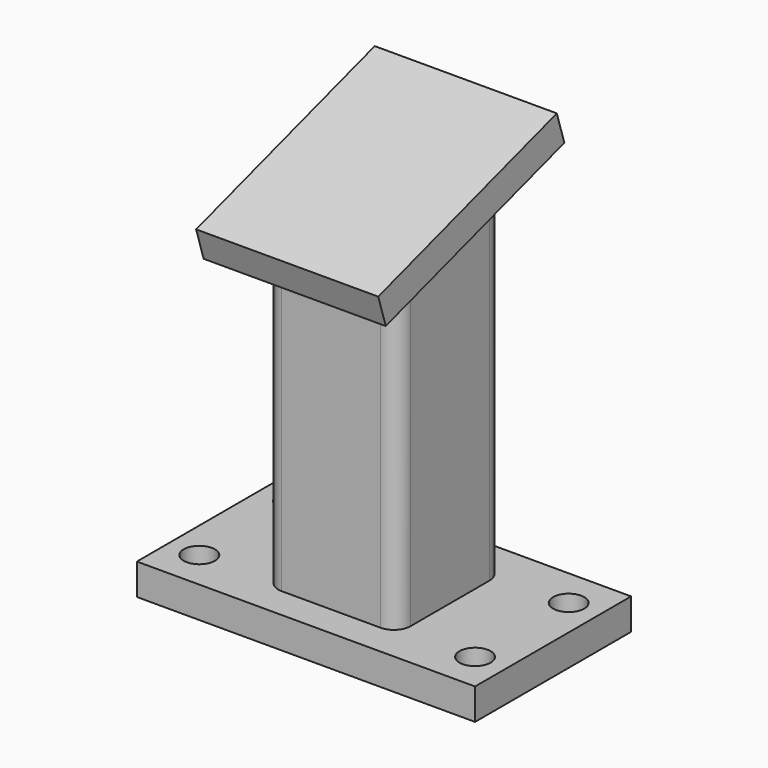
from build123d import *

# Parameters (mm, degrees)
F0_W     = 130
F0_H     = 75
F1_DEPTH = 12
F3_DEPTH = 136
F5_D     = 12
F7_DEPTH = 50.8
F8_W     = 70
F8_H     = 90
F9_DEPTH = 12


with BuildPart() as f1:
    # F0 (on Top) → F1 (new body)
    with BuildSketch(Plane.XY):
        Rectangle(F0_W, F0_H)
    extrude(amount=-F1_DEPTH)

    # F2 (on face) → F3 (join)
    with BuildSketch(Plane.XY):
        with BuildLine():
            Line((-19.05, -25.4), (19.05, -25.4))
            ThreePointArc((19.05, -25.4), (23.5401280605, -23.5401280605), (25.4, -19.05))
            Line((25.4, -19.05), (25.4, 19.05))
            ThreePointArc((25.4, 19.05), (23.5401280605, 23.5401280605), (19.05, 25.4))
            Line((19.05, 25.4), (-19.05, 25.4))
            ThreePointArc((-19.05, 25.4), (-23.5401280605, 23.5401280605), (-25.4, 19.05))
            Line((-25.4, 19.05), (-25.4, -19.05))
            ThreePointArc((-25.4, -19.05), (-23.5401280605, -23.5401280605), (-19.05, -25.4))
        make_face()
        with BuildLine():
            Line((-12.7, 19.05), (12.7, 19.05))
            ThreePointArc((12.7, 19.05), (17.1901280605, 17.1901280605), (19.05, 12.7))
            Line((19.05, 12.7), (19.05, -12.7))
            ThreePointArc((19.05, -12.7), (17.1901280605, -17.1901280605), (12.7, -19.05))
            Line((12.7, -19.05), (-12.7, -19.05))
            ThreePointArc((-12.7, -19.05), (-17.1901280605, -17.1901280605), (-19.05, -12.7))
            Line((-19.05, -12.7), (-19.05, 12.7))
            ThreePointArc((-19.05, 12.7), (-17.1901280605, 17.1901280605), (-12.7, 19.05))
        make_face(mode=Mode.SUBTRACT)
    extrude(amount=F3_DEPTH)

    # F5 (through all)
    with Locations(Plane.XY):
        with Locations((-53, 22.5), (53, 22.5), (53, -22.5), (-53, -22.5)):
            Hole(F5_D / 2)

    # F6 (on face) → F7 (cut)
    with BuildSketch(Plane.YZ.offset(25.4)):
        Polygon((-19.05, 136), (-25.4, 136), (-25.4, 119.9340696072), (-19.05, 121.9423109063), align=None)
        Polygon((19.05, 136), (-19.05, 136), (-19.05, 121.9423109063), (19.05, 133.9917587009), align=None)
        Polygon((25.4, 136), (19.05, 136), (19.05, 133.9917587009), align=None)
    extrude(amount=-F7_DEPTH, mode=Mode.SUBTRACT)

    # F8 (on face) → F9 (join)
    with BuildSketch(Plane(origin=(0, -36.7908585502, 116.331614084), x_dir=(1, 0, 0), z_dir=(0, -0.3015379599, 0.9534541723))):
        with Locations((0, 38.5869186148)):
            Rectangle(F8_W, F8_H)
        with BuildLine():
            Line((25.4, 58.5669035507), (25.4, 18.6069336789))
            add(Edge.make_bspline(
                [(25.4, 18.6069336789), (25.4, 11.9469387003), (19.05, 11.9469387003)],
                knots=[4.7123889804, 4.7123889804, 4.7123889804, 6.2831853072, 6.2831853072, 6.2831853072], degree=2, weights=[1, 0.7071067812, 1]))
            Line((19.05, 11.9469387003), (-19.05, 11.9469387003))
            add(Edge.make_bspline(
                [(-19.05, 11.9469387003), (-25.4, 11.9469387003), (-25.4, 18.6069336789)],
                knots=[0, 0, 0, 1.5707963268, 1.5707963268, 1.5707963268], degree=2, weights=[1, 0.7071067812, 1]))
            Line((-25.4, 18.6069336789), (-25.4, 58.5669035507))
            add(Edge.make_bspline(
                [(-25.4, 58.5669035507), (-25.4, 65.2268985294), (-19.05, 65.2268985294)],
                knots=[1.5707963268, 1.5707963268, 1.5707963268, 3.1415926536, 3.1415926536, 3.1415926536], degree=2, weights=[1, 0.7071067812, 1]))
            Line((-19.05, 65.2268985294), (19.05, 65.2268985294))
            add(Edge.make_bspline(
                [(19.05, 65.2268985294), (25.4, 65.2268985294), (25.4, 58.5669035507)],
                knots=[3.1415926536, 3.1415926536, 3.1415926536, 4.7123889804, 4.7123889804, 4.7123889804], degree=2, weights=[1, 0.7071067812, 1]))
        make_face(mode=Mode.SUBTRACT)
        with BuildLine():
            add(Edge.make_bspline(
                [(25.4, 18.6069336789), (25.4, 11.9469387003), (19.05, 11.9469387003)],
                knots=[4.7123889804, 4.7123889804, 4.7123889804, 6.2831853072, 6.2831853072, 6.2831853072], degree=2, weights=[1, 0.7071067812, 1]))
            Line((25.4, 18.6069336789), (25.4, 58.5669035507))
            add(Edge.make_bspline(
                [(19.05, 65.2268985294), (25.4, 65.2268985294), (25.4, 58.5669035507)],
                knots=[3.1415926536, 3.1415926536, 3.1415926536, 4.7123889804, 4.7123889804, 4.7123889804], degree=2, weights=[1, 0.7071067812, 1]))
            Line((19.05, 65.2268985294), (-19.05, 65.2268985294))
            add(Edge.make_bspline(
                [(-25.4, 58.5669035507), (-25.4, 65.2268985294), (-19.05, 65.2268985294)],
                knots=[1.5707963268, 1.5707963268, 1.5707963268, 3.1415926536, 3.1415926536, 3.1415926536], degree=2, weights=[1, 0.7071067812, 1]))
            Line((-25.4, 58.5669035507), (-25.4, 18.6069336789))
            add(Edge.make_bspline(
                [(-19.05, 11.9469387003), (-25.4, 11.9469387003), (-25.4, 18.6069336789)],
                knots=[0, 0, 0, 1.5707963268, 1.5707963268, 1.5707963268], degree=2, weights=[1, 0.7071067812, 1]))
            Line((-19.05, 11.9469387003), (19.05, 11.9469387003))
        make_face()
        with BuildLine():
            Line((-19.05, 25.2669286576), (-19.05, 51.9069085721))
            add(Edge.make_bspline(
                [(-19.05, 51.9069085721), (-19.05, 58.5669035507), (-12.7, 58.5669035507)],
                knots=[1.5707963268, 1.5707963268, 1.5707963268, 3.1415926536, 3.1415926536, 3.1415926536], degree=2, weights=[1, 0.7071067812, 1]))
            Line((-12.7, 58.5669035507), (12.7, 58.5669035507))
            add(Edge.make_bspline(
                [(12.7, 58.5669035507), (19.05, 58.5669035507), (19.05, 51.9069085721)],
                knots=[3.1415926536, 3.1415926536, 3.1415926536, 4.7123889804, 4.7123889804, 4.7123889804], degree=2, weights=[1, 0.7071067812, 1]))
            Line((19.05, 51.9069085721), (19.05, 25.2669286576))
            add(Edge.make_bspline(
                [(19.05, 25.2669286576), (19.05, 18.6069336789), (12.7, 18.6069336789)],
                knots=[4.7123889804, 4.7123889804, 4.7123889804, 6.2831853072, 6.2831853072, 6.2831853072], degree=2, weights=[1, 0.7071067812, 1]))
            Line((12.7, 18.6069336789), (-12.7, 18.6069336789))
            add(Edge.make_bspline(
                [(-12.7, 18.6069336789), (-19.05, 18.6069336789), (-19.05, 25.2669286576)],
                knots=[0, 0, 0, 1.5707963268, 1.5707963268, 1.5707963268], degree=2, weights=[1, 0.7071067812, 1]))
        make_face(mode=Mode.SUBTRACT)
        with BuildLine():
            add(Edge.make_bspline(
                [(-19.05, 51.9069085721), (-19.05, 58.5669035507), (-12.7, 58.5669035507)],
                knots=[1.5707963268, 1.5707963268, 1.5707963268, 3.1415926536, 3.1415926536, 3.1415926536], degree=2, weights=[1, 0.7071067812, 1]))
            Line((-19.05, 51.9069085721), (-19.05, 25.2669286576))
            add(Edge.make_bspline(
                [(-12.7, 18.6069336789), (-19.05, 18.6069336789), (-19.05, 25.2669286576)],
                knots=[0, 0, 0, 1.5707963268, 1.5707963268, 1.5707963268], degree=2, weights=[1, 0.7071067812, 1]))
            Line((-12.7, 18.6069336789), (12.7, 18.6069336789))
            add(Edge.make_bspline(
                [(19.05, 25.2669286576), (19.05, 18.6069336789), (12.7, 18.6069336789)],
                knots=[4.7123889804, 4.7123889804, 4.7123889804, 6.2831853072, 6.2831853072, 6.2831853072], degree=2, weights=[1, 0.7071067812, 1]))
            Line((19.05, 25.2669286576), (19.05, 51.9069085721))
            add(Edge.make_bspline(
                [(12.7, 58.5669035507), (19.05, 58.5669035507), (19.05, 51.9069085721)],
                knots=[3.1415926536, 3.1415926536, 3.1415926536, 4.7123889804, 4.7123889804, 4.7123889804], degree=2, weights=[1, 0.7071067812, 1]))
            Line((12.7, 58.5669035507), (-12.7, 58.5669035507))
        make_face()
    extrude(amount=F9_DEPTH)


solid = f1.part
